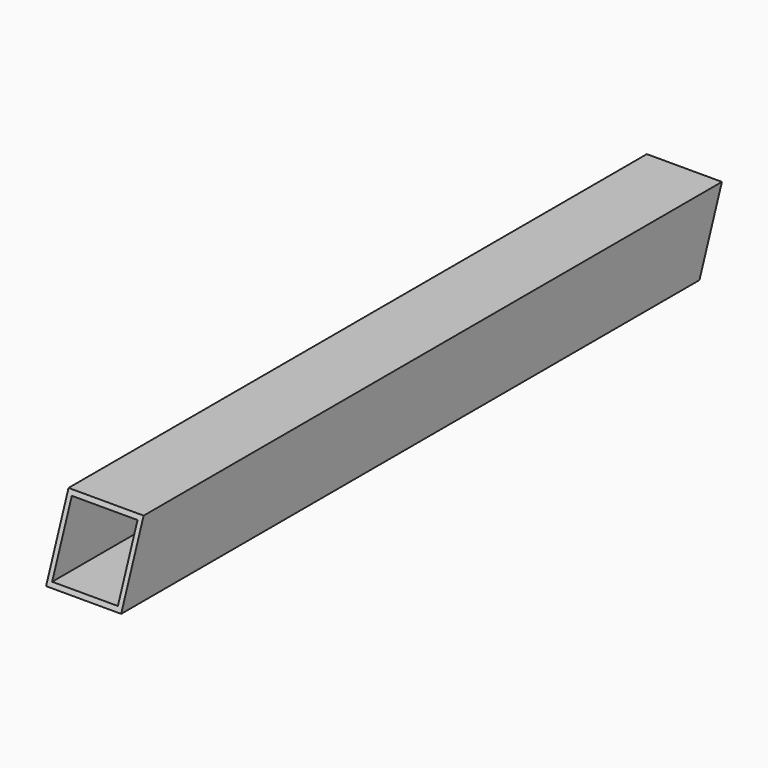
from build123d import *

# Parameters (mm, degrees)
F0_W        = 25.4
F0_H        = 25.4
F0_W_2      = 22.225
F0_H_2      = 22.225
F1_DEPTH    = 254
F2_T1_DEPTH = 157.170304922
F3_T1_DEPTH = 157.170304922


# Not quite as in the source:
# - a fillet or chamfer that OpenCascade refuses, or shapes differently, is made with other operations: its cross-section is extruded or revolved along the edge and cut away or added


with BuildPart() as f1:
    # F0 (on Front) → F1 (new body)
    with BuildSketch(Plane.XZ):
        Rectangle(F0_W, F0_H)
        Rectangle(F0_W_2, F0_H_2, mode=Mode.SUBTRACT)
    extrude(amount=F1_DEPTH)

    # F2: chamfer of 25.4 x 9.4966708589 on 1 edges, made by hand

    # F2_s2 → F2_t1 (cut)
    with BuildSketch(Plane.YZ.offset(-78.585152461)):
        Polygon((-244.5033291411, 12.7), (-254, -12.7), (-254, 12.7), align=None)
    extrude(amount=F2_T1_DEPTH, mode=Mode.SUBTRACT)

    # F3: chamfer of 25.4 x 9.4966708589 on 1 edges, made by hand

    # F3_s2 → F3_t1 (cut)
    with BuildSketch(Plane.YZ.offset(-78.585152461)):
        Polygon((0, 12.7), (-9.4966708589, -12.7), (0, -12.7), align=None)
    extrude(amount=F3_T1_DEPTH, mode=Mode.SUBTRACT)


solid = f1.part
